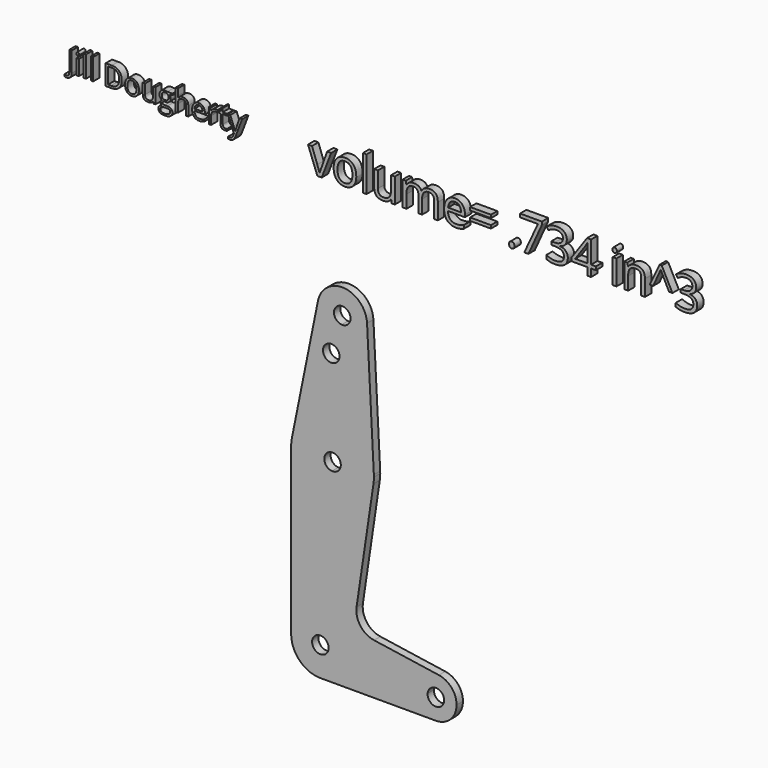
from build123d import *

# Parameters (mm, degrees)
F0_TEXT_SIZE   = 10.8186155558
F0_TEXT_SIZE_2 = 17.6572758291
F1_DEPTH       = 3.048


# Not quite as in the source:
# - Text() gives the source's letters only with a copy of the font that has no kerning and outlines rounded to 1/6400 em; it was checked with that copy


with BuildPart() as f1:
    # F0 (on Front) → F1 (new body)
    with BuildSketch(Plane.XZ):
        with BuildLine():
            ThreePointArc((3.1664054306, -0.2334558824), (-2.4040649895, -2.0739085145), (0.2334558824, 3.1664054306))
            Line((0.2334558824, 3.1664054306), (0.8239619377, 11.1755485786))
            ThreePointArc((0.8239619377, 11.1755485786), (-7.6268794002, 8.2099031616), (-11.2058823529, 0))
            ThreePointArc((-11.2058823529, 0), (-7.9237554009, -7.9237554009), (0, -11.2058823529))
            ThreePointArc((0, -11.2058823529), (7.6268794002, -8.2099031616), (11.1755485786, -0.8239619377))
            Line((11.1755485786, -0.8239619377), (3.1664054306, -0.2334558824))
        make_face()
        with BuildLine():
            ThreePointArc((-11.2058823529, 0), (-7.6268794002, 8.2099031616), (0.8239619377, 11.1755485786))
            Line((0.8239619377, 11.1755485786), (3.5018382353, 47.4960814591))
            ThreePointArc((3.5018382353, 47.4960814591), (-6.9615784985, 52.5233627952), (-11.2058823529, 63.3281086122))
            Line((-11.2058823529, 63.3281086122), (-11.2058823529, 0))
        make_face()
        with BuildLine():
            Line((3.5018382353, 47.4960814591), (0.8239619377, 11.1755485786))
            ThreePointArc((0.8239619377, 11.1755485786), (8.2099031616, 7.6268794002), (11.2058823529, 0))
            ThreePointArc((11.2058823529, 0), (11.1982963416, -0.4122600553), (11.1755485786, -0.8239619377))
            Line((11.1755485786, -0.8239619377), (36.413662452, -2.6847426471))
            ThreePointArc((36.413662452, -2.6847426471), (39.3695262017, 2.9284571597), (45.4937956721, 4.5832882785))
            Line((45.4937956721, 4.5832882785), (20.5924078105, 8.2752662184))
            ThreePointArc((20.5924078105, 8.2752662184), (15.373063402, 11.4031207696), (13.8941567411, 17.305481758))
            Line((13.8941567411, 17.305481758), (20.37245891, 60.999869325))
            ThreePointArc((20.37245891, 60.999869325), (14.5894173006, 50.9344295869), (3.5018382353, 47.4960814591))
        make_face()
        with BuildLine():
            Line((36.413662452, -2.6847426471), (11.1755485786, -0.8239619377))
            ThreePointArc((11.1755485786, -0.8239619377), (7.6268794002, -8.2099031616), (0, -11.2058823529))
            Line((0, -11.2058823529), (44.3296760285, -11.2058823529))
            ThreePointArc((44.3296760285, -11.2058823529), (38.5143279557, -8.6707552614), (36.413662452, -2.6847426471))
        make_face()
        with BuildLine():
            ThreePointArc((-11.2058823529, 63.3281086122), (-6.9615784985, 52.5233627952), (3.5018382353, 47.4960814591))
            Line((3.5018382353, 47.4960814591), (4.4356617647, 60.1617031816))
            ThreePointArc((4.4356617647, 60.1617031816), (1.5027122164, 63.5615644945), (4.9025735294, 66.4945140428))
            Line((4.9025735294, 66.4945140428), (5.8363970588, 79.1601357652))
            ThreePointArc((5.8363970588, 79.1601357652), (-4.9273244434, 75.9742117355), (-10.8928249003, 66.4652361441))
            ThreePointArc((-10.8928249003, 66.4652361441), (-11.1274241096, 64.9044631186), (-11.2058823529, 63.3281086122))
        make_face()
        with BuildLine():
            Line((4.4356617647, 60.1617031816), (3.5018382353, 47.4960814591))
            ThreePointArc((3.5018382353, 47.4960814591), (14.5894173006, 50.9344295869), (20.37245891, 60.999869325))
            ThreePointArc((20.37245891, 60.999869325), (20.5011448001, 62.1608292004), (20.5441176471, 63.3281086122))
            ThreePointArc((20.5441176471, 63.3281086122), (20.538807359, 63.738685581), (20.5228800474, 64.1489878686))
            ThreePointArc((20.5228800474, 64.1489878686), (16.0164788551, 74.4300462185), (5.8363970588, 79.1601357652))
            Line((5.8363970588, 79.1601357652), (4.9025735294, 66.4945140428))
            ThreePointArc((4.9025735294, 66.4945140428), (6.9952568762, 65.4890577756), (7.8441176471, 63.3281086122))
            ThreePointArc((7.8441176471, 63.3281086122), (6.8300668105, 61.0019693831), (4.4356617647, 60.1617031816))
        make_face()
        with BuildLine():
            ThreePointArc((45.4937956721, 4.5832882785), (39.3695262017, 2.9284571597), (36.413662452, -2.6847426471))
            ThreePointArc((36.413662452, -2.6847426471), (38.5143279557, -8.6707552614), (44.3296760285, -11.2058823529))
            ThreePointArc((44.3296760285, -11.2058823529), (49.9423361042, -8.8810424286), (52.2671760285, -3.2683823529))
            ThreePointArc((52.2671760285, -3.2683823529), (50.3398385023, 1.9163889332), (45.4937956721, 4.5832882785))
        make_face()
        with BuildLine():
            ThreePointArc((47.5046760285, -3.2683823529), (44.2128690129, -6.4412329831), (41.1632705979, -3.0349264706))
            ThreePointArc((41.1632705979, -3.0349264706), (44.4464830442, -0.0955317228), (47.5046760285, -3.2683823529))
        make_face(mode=Mode.SUBTRACT)
        with BuildLine():
            Line((-0.9327537637, 115.8728720211), (-10.8928249003, 66.4652361441))
            ThreePointArc((-10.8928249003, 66.4652361441), (-4.9273244434, 75.9742117355), (5.8363970588, 79.1601357652))
            Line((5.8363970588, 79.1601357652), (7.344871375, 99.619852687))
            Line((7.344871375, 99.619852687), (7.7040441176, 104.4913792101))
            ThreePointArc((7.7040441176, 104.4913792101), (0.8167498907, 108.2327302477), (-0.9327537637, 115.8728720211))
        make_face()
        with BuildLine():
            ThreePointArc((7.3534659475, 99.8533086122), (7.3513165769, 99.7365015751), (7.344871375, 99.619852687))
            ThreePointArc((7.344871375, 99.619852687), (1.0056153182, 99.9701156493), (7.3534659475, 99.8533086122))
        make_face(mode=Mode.SUBTRACT)
        with BuildLine():
            Line((7.344871375, 99.619852687), (5.8363970588, 79.1601357652))
            ThreePointArc((5.8363970588, 79.1601357652), (16.0164788551, 74.4300462185), (20.5228800474, 64.1489878686))
            Line((20.5228800474, 64.1489878686), (17.9166692049, 114.4831230558))
            ThreePointArc((17.9166692049, 114.4831230558), (17.9262255919, 114.2369416832), (17.9294117647, 113.990595502))
            ThreePointArc((17.9294117647, 113.990595502), (14.8872592549, 107.0121778146), (7.7040441176, 104.4913792101))
            Line((7.7040441176, 104.4913792101), (7.344871375, 99.619852687))
        make_face()
        with BuildLine():
            ThreePointArc((17.9166692049, 114.4831230558), (9.1047794118, 123.4898117938), (-0.9327537637, 115.8728720211))
            ThreePointArc((-0.9327537637, 115.8728720211), (0.8167498907, 108.2327302477), (7.7040441176, 104.4913792101))
            ThreePointArc((7.7040441176, 104.4913792101), (14.8872592549, 107.0121778146), (17.9294117647, 113.990595502))
            ThreePointArc((17.9294117647, 113.990595502), (17.9262255919, 114.2369416832), (17.9166692049, 114.4831230558))
        make_face()
        with BuildLine():
            ThreePointArc((11.5794117647, 113.990595502), (10.5653609281, 111.6644562728), (8.1709558824, 110.8241900713))
            ThreePointArc((8.1709558824, 110.8241900713), (6.2434626013, 116.3167347311), (11.5794117647, 113.990595502))
        make_face(mode=Mode.SUBTRACT)
        with Locations((-97.3515734076, 161.9699448347)):
            Text('Jill Dougherty', F0_TEXT_SIZE, font='Open Sans', text_align=(TextAlign.LEFT, TextAlign.BOTTOM))
        with Locations((-4.7367289662, 158.021941781)):
            Text('volume= .734 in^3', F0_TEXT_SIZE_2, font='Open Sans', text_align=(TextAlign.LEFT, TextAlign.BOTTOM))
        with BuildLine():
            Line((0.8239619377, 11.1755485786), (0.2334558824, 3.1664054306))
            ThreePointArc((0.2334558824, 3.1664054306), (2.3261392291, 2.1609491634), (3.175, 0))
            ThreePointArc((3.175, 0), (3.1728506301, -0.1168070157), (3.1664054306, -0.2334558824))
            Line((3.1664054306, -0.2334558824), (11.1755485786, -0.8239619377))
            ThreePointArc((11.1755485786, -0.8239619377), (11.1982963416, -0.4122600553), (11.2058823529, 0))
            ThreePointArc((11.2058823529, 0), (8.2099031616, 7.6268794002), (0.8239619377, 11.1755485786))
        make_face()
    extrude(amount=F1_DEPTH)


solid = f1.part
